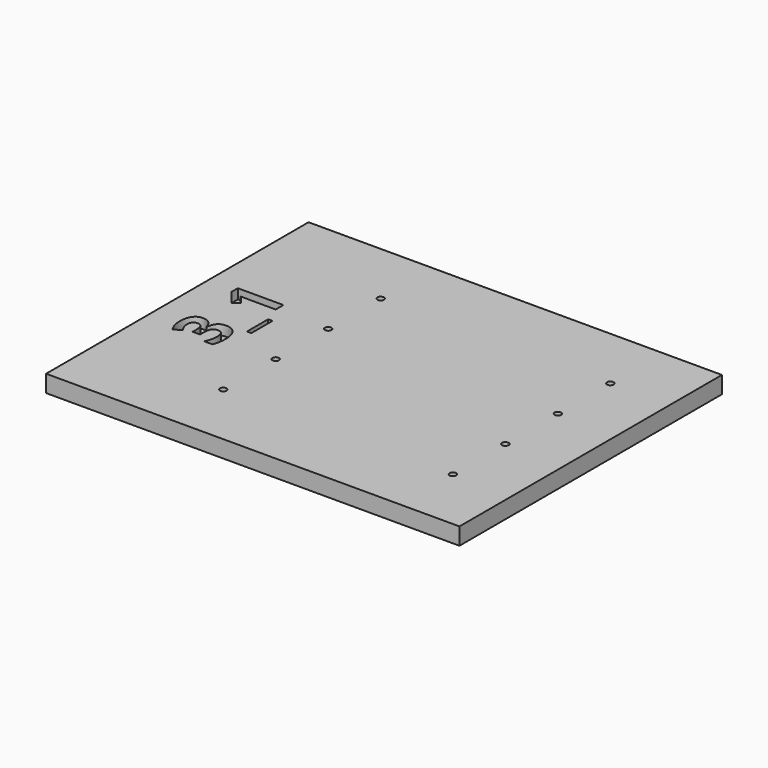
from build123d import *

# Parameters (mm, degrees)
F0_W         = 63
F0_H         = 50
F1_DEPTH     = 2.6
F2_TEXT_SIZE = 9.7222222222
F3_DEPTH     = 1.5
F4_R         = 0.5
F5_DEPTH     = 2.6


# Not quite as in the source:
# - Text() gives the source's letters only with a copy of the font that has no kerning and outlines rounded to 1/6400 em; it was checked with that copy


with BuildPart() as f1:
    # F0 (on Top) → F1 (new body)
    with BuildSketch(Plane.XY):
        with Locations((-11.6587231159, 3.3350909071)):
            Rectangle(F0_W, F0_H)
    extrude(amount=F1_DEPTH)

    # F2 (on face) → F3 (cut)
    with BuildSketch(Plane.XY.offset(2.6)):
        with Locations(Location((-32.1587231159, -3.7649090929), (0, 0, 90))):
            Text('3_1', F2_TEXT_SIZE, font='Open Sans', font_style=FontStyle.BOLD, text_align=(TextAlign.LEFT, TextAlign.BOTTOM))
    extrude(amount=-F3_DEPTH, mode=Mode.SUBTRACT)

    # F4 (on face) → F5 (cut, through all)
    with BuildSketch(Plane.XY.offset(2.6)):
        with Locations((-24.1587231159, -11.6649090929)):
            Circle(F4_R)
        with Locations((-24.1587231159, -1.6649090929)):
            Circle(F4_R)
        with Locations((-24.1587231159, 8.3350909071)):
            Circle(F4_R)
        with Locations((-24.1587231159, 18.3350909071)):
            Circle(F4_R)
        with Locations((10.8412768841, -11.6649090929)):
            Circle(F4_R)
        with Locations((10.8412768841, -1.6649090929)):
            Circle(F4_R)
        with Locations((10.8412768841, 8.3350909071)):
            Circle(F4_R)
        with Locations((10.8412768841, 18.3350909071)):
            Circle(F4_R)
    extrude(amount=-F5_DEPTH, mode=Mode.SUBTRACT)


solid = f1.part
